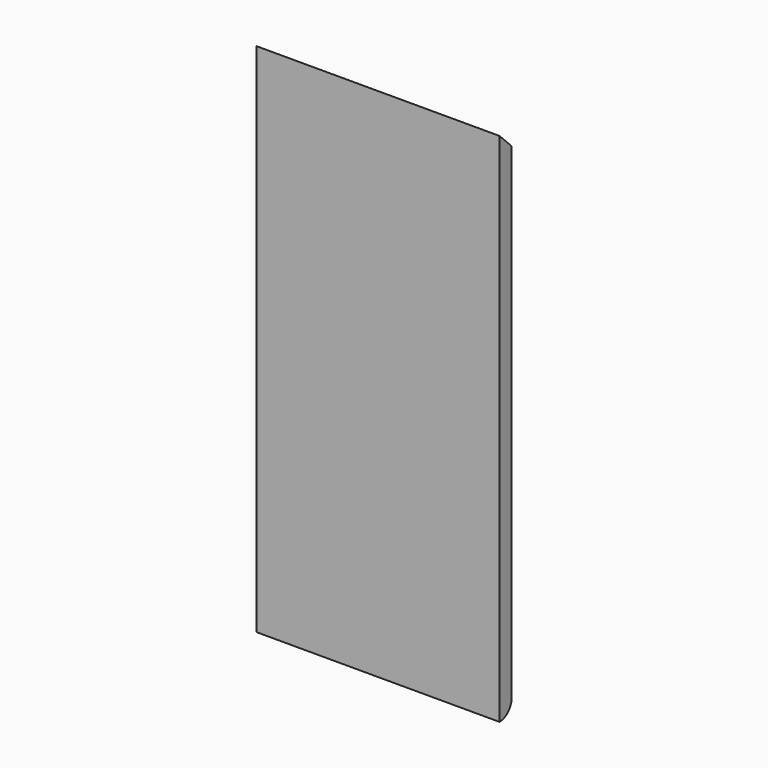
from build123d import *

# Parameters (mm, degrees)
F0_W     = 80
F0_H     = 169.70563
F1_DEPTH = 5
F2_SIZE  = 4.99999
F3_R     = 4.99999


# Not quite as in the source:
# - a fillet or chamfer is up to 0.001 mm smaller than in the source, because OpenCascade refuses the exact size


with BuildPart() as f1:
    # F0 (on Front) → F1 (new body)
    with BuildSketch(Plane.XZ):
        with Locations((-37.0779657288, 20.5572328247)):
            Rectangle(F0_W, F0_H)
    extrude(amount=F1_DEPTH)

    # F2 (size 5 in the source; OpenCascade refuses exactly that, so slightly less here)
    f2_edges = [f1.edges().sort_by_distance(p)[0] for p in [
        (-37.077966, 0, 105.410048),
    ]]
    chamfer(f2_edges, length=F2_SIZE)

    # F3 (radius 5 in the source; OpenCascade refuses exactly that, so slightly less here)
    f3_edges = [f1.edges().sort_by_distance(p)[0] for p in [
        (-37.077966, 0, -64.295582),
    ]]
    fillet(f3_edges, radius=F3_R)


solid = f1.part
